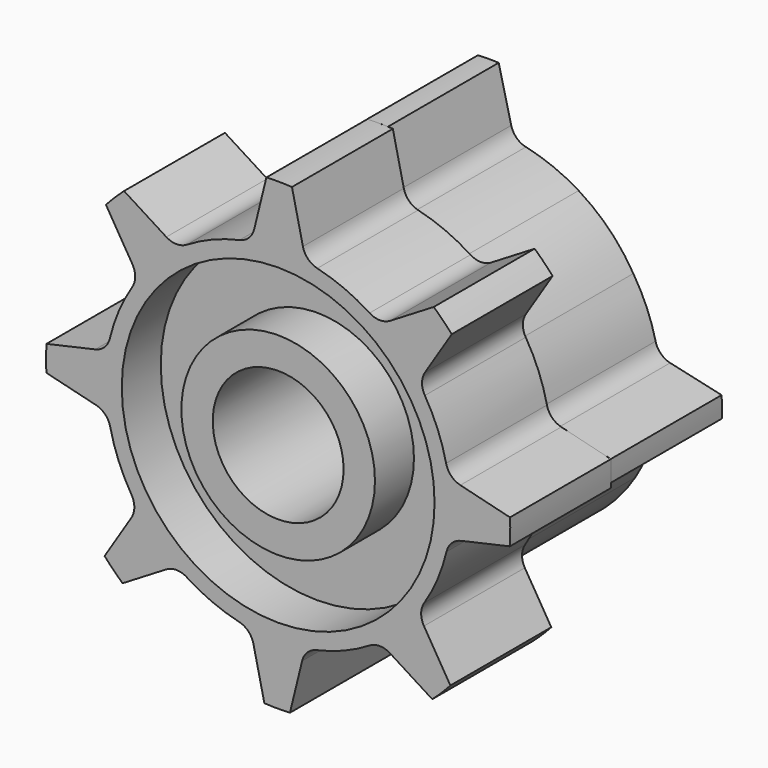
from build123d import *

# Parameters (mm, degrees)
F0_R     = 76.2109388573
F0_R_2   = 51.3540335205
F1_DEPTH = 41.402
F0_R_3   = 31.7840451581
F0_R_4   = 21.4823406774
F2_DEPTH = 25.4
F4_DEPTH = 71.882
F5_DEPTH = 45.466
F6_DEPTH = 31.496
F8_DEPTH = 51.054


with BuildPart() as f1:
    # F0 (on Front) → F1 (new body)
    with BuildSketch(Plane.XZ):
        Circle(F0_R)
        Circle(F0_R_2, mode=Mode.SUBTRACT)
    extrude(amount=F1_DEPTH)

    # F3 (on face) → F4 (cut)
    with BuildSketch(Plane.XZ.offset(41.402)):
        with BuildLine():
            Line((-47.8672647572, 36.7388077798), (-56.5527223926, 51.0871489857))
            ThreePointArc((-56.5527223926, 51.0871489857), (-70.2816834344, 29.4718878788), (-76.0762226062, 4.529410059))
            Line((-76.0762226062, 4.529410059), (-60.0498225812, 8.1337879145))
            ThreePointArc((-60.0498225812, 8.1337879145), (-56.9862917555, 9.8058862302), (-55.2691454533, 12.8443961405))
            ThreePointArc((-55.2691454533, 12.8443961405), (-52.3275453278, 21.741673907), (-47.9509285541, 30.0277941433))
            ThreePointArc((-47.9509285541, 30.0277941433), (-46.9500267793, 33.3713445818), (-47.8672647572, 36.7388077798))
        make_face()
        with BuildLine():
            Line((-7.8690073929, 59.8255276205), (-3.8647440191, 76.1128829777))
            ThreePointArc((-3.8647440191, 76.1128829777), (-28.8568831762, 70.5364267231), (-50.5912363244, 56.9967894593))
            Line((-50.5912363244, 56.9967894593), (-36.7101801652, 48.2130933472))
            ThreePointArc((-36.7101801652, 48.2130933472), (-33.361584686, 47.2292019839), (-29.9988279292, 48.1635471516))
            ThreePointArc((-29.9988279292, 48.1635471516), (-21.6274770901, 52.3748471981), (-12.673569882, 55.1392836076))
            ThreePointArc((-12.673569882, 55.1392836076), (-9.6015782614, 56.7957863637), (-7.8690073929, 59.8255276205))
        make_face()
        with BuildLine():
            ThreePointArc((51.0871489857, 56.5527223926), (29.4718878788, 70.2816834344), (4.529410059, 76.0762226062))
            Line((4.529410059, 76.0762226062), (8.1337879145, 60.0498225812))
            ThreePointArc((8.1337879145, 60.0498225812), (9.8058862302, 56.9862917555), (12.8443961405, 55.2691454533))
            ThreePointArc((12.8443961405, 55.2691454533), (21.741673907, 52.3275453278), (30.0277941433, 47.9509285541))
            ThreePointArc((30.0277941433, 47.9509285541), (33.3713445818, 46.9500267793), (36.7388077798, 47.8672647572))
            Line((36.7388077798, 47.8672647572), (51.0871489857, 56.5527223926))
        make_face()
        with BuildLine():
            ThreePointArc((76.1128829777, 3.8647440191), (70.5364267231, 28.8568831762), (56.9967894593, 50.5912363244))
            Line((56.9967894593, 50.5912363244), (48.2130933472, 36.7101801652))
            ThreePointArc((48.2130933472, 36.7101801652), (47.2292019839, 33.361584686), (48.1635471516, 29.9988279292))
            ThreePointArc((48.1635471516, 29.9988279292), (52.3748471981, 21.6274770901), (55.1392836076, 12.673569882))
            ThreePointArc((55.1392836076, 12.673569882), (56.7957863637, 9.6015782614), (59.8255276205, 7.8690073929))
            Line((59.8255276205, 7.8690073929), (76.1128829777, 3.8647440191))
        make_face()
        with BuildLine():
            ThreePointArc((56.5527223926, -51.0871489857), (70.2816834344, -29.4718878788), (76.0762226062, -4.529410059))
            Line((76.0762226062, -4.529410059), (60.0498225812, -8.1337879145))
            ThreePointArc((60.0498225812, -8.1337879145), (56.9862917555, -9.8058862302), (55.2691454533, -12.8443961405))
            ThreePointArc((55.2691454533, -12.8443961405), (52.3275453278, -21.741673907), (47.9509285541, -30.0277941433))
            ThreePointArc((47.9509285541, -30.0277941433), (46.9500267793, -33.3713445818), (47.8672647572, -36.7388077798))
            Line((47.8672647572, -36.7388077798), (56.5527223926, -51.0871489857))
        make_face()
        with BuildLine():
            ThreePointArc((3.8647440191, -76.1128829777), (28.8568831762, -70.5364267231), (50.5912363244, -56.9967894593))
            Line((50.5912363244, -56.9967894593), (36.7101801652, -48.2130933472))
            ThreePointArc((36.7101801652, -48.2130933472), (33.361584686, -47.2292019839), (29.9988279292, -48.1635471516))
            ThreePointArc((29.9988279292, -48.1635471516), (21.6274770901, -52.3748471981), (12.673569882, -55.1392836076))
            ThreePointArc((12.673569882, -55.1392836076), (9.6015782614, -56.7957863637), (7.8690073929, -59.8255276205))
            Line((7.8690073929, -59.8255276205), (3.8647440191, -76.1128829777))
        make_face()
        with BuildLine():
            Line((-36.7388077798, -47.8672647572), (-51.0871489857, -56.5527223926))
            ThreePointArc((-51.0871489857, -56.5527223926), (-29.4718878788, -70.2816834344), (-4.529410059, -76.0762226062))
            Line((-4.529410059, -76.0762226062), (-8.1337879145, -60.0498225812))
            ThreePointArc((-8.1337879145, -60.0498225812), (-9.8058862302, -56.9862917555), (-12.8443961405, -55.2691454533))
            ThreePointArc((-12.8443961405, -55.2691454533), (-21.741673907, -52.3275453278), (-30.0277941433, -47.9509285541))
            ThreePointArc((-30.0277941433, -47.9509285541), (-33.3713445818, -46.9500267793), (-36.7388077798, -47.8672647572))
        make_face()
        with BuildLine():
            Line((-59.8255276205, -7.8690073929), (-76.1128829777, -3.8647440191))
            ThreePointArc((-76.1128829777, -3.8647440191), (-70.5364267231, -28.8568831762), (-56.9967894593, -50.5912363244))
            Line((-56.9967894593, -50.5912363244), (-48.2130933472, -36.7101801652))
            ThreePointArc((-48.2130933472, -36.7101801652), (-47.2292019839, -33.361584686), (-48.1635471516, -29.9988279292))
            ThreePointArc((-48.1635471516, -29.9988279292), (-52.3748471981, -21.6274770901), (-55.1392836076, -12.673569882))
            ThreePointArc((-55.1392836076, -12.673569882), (-56.7957863637, -9.6015782614), (-59.8255276205, -7.8690073929))
        make_face()
    extrude(amount=-F4_DEPTH, mode=Mode.SUBTRACT)


with BuildPart() as f1b:
    # F0 (on Front) → F1, piece 2 (new body)
    with BuildSketch(Plane.XZ):
        Circle(F0_R_3)
        Circle(F0_R_4, mode=Mode.SUBTRACT)
    extrude(amount=F1_DEPTH)


with BuildPart() as f2:
    # F0 (on Front) → F2 (new body)
    with BuildSketch(Plane.XZ):
        Circle(F0_R_2)
        Circle(F0_R_3, mode=Mode.SUBTRACT)
    extrude(amount=F2_DEPTH)


with BuildPart() as f5:
    # F0 (on Front) → F5 (new body)
    with BuildSketch(Plane.XZ):
        Circle(F0_R_3)
        Circle(F0_R_4, mode=Mode.SUBTRACT)
    extrude(amount=-F5_DEPTH)


with BuildPart() as f5b:
    # F0 (on Front) → F5, piece 2 (new body)
    with BuildSketch(Plane.XZ):
        Circle(F0_R)
        Circle(F0_R_2, mode=Mode.SUBTRACT)
    extrude(amount=-F5_DEPTH)

    # F7 (on face) → F8 (cut)
    with BuildSketch(Plane(origin=(0, 45.466, 0), x_dir=(-1, 0, 0), z_dir=(0, 1, 0))):
        with BuildLine():
            ThreePointArc((-47.1182366423, 29.5992543095), (-39.2509800473, 39.7646962899), (-29.1661360175, 47.7350073178))
            ThreePointArc((-29.1661360175, 47.7350073178), (-20.7947851783, 51.9463073643), (-11.8408779702, 54.7107437738))
            ThreePointArc((-11.8408779702, 54.7107437738), (-8.7688863497, 56.3672465299), (-7.0363154811, 59.3969877867))
            Line((-7.0363154811, 59.3969877867), (-2.9163110774, 76.1551201903))
            ThreePointArc((-2.9163110774, 76.1551201903), (-53.5379377777, 54.2383298048), (-76.1107860532, 3.9058223039))
            Line((-76.1107860532, 3.9058223039), (-59.2171306694, 7.7052480807))
            ThreePointArc((-59.2171306694, 7.7052480807), (-56.1535998437, 9.3773463964), (-54.4364535416, 12.4158563067))
            ThreePointArc((-54.4364535416, 12.4158563067), (-51.494853416, 21.3131340732), (-47.1182366423, 29.5992543095))
        make_face()
        with BuildLine():
            ThreePointArc((76.1551201903, 2.9163110774), (54.2383298048, 53.5379377777), (3.9058223039, 76.1107860532))
            Line((3.9058223039, 76.1107860532), (7.7052480807, 59.2171306694))
            ThreePointArc((7.7052480807, 59.2171306694), (9.3773463964, 56.1535998437), (12.4158563067, 54.4364535416))
            ThreePointArc((12.4158563067, 54.4364535416), (21.3131340732, 51.494853416), (29.5992543095, 47.1182366423))
            ThreePointArc((29.5992543095, 47.1182366423), (39.7646962899, 39.2509800473), (47.7350073178, 29.1661360175))
            ThreePointArc((47.7350073178, 29.1661360175), (51.9463073643, 20.7947851783), (54.7107437738, 11.8408779702))
            ThreePointArc((54.7107437738, 11.8408779702), (56.3672465299, 8.7688863497), (59.3969877867, 7.0363154811))
            Line((59.3969877867, 7.0363154811), (76.1551201903, 2.9163110774))
        make_face()
        with BuildLine():
            ThreePointArc((2.9163110774, -76.1551201903), (53.5379377777, -54.2383298048), (76.1107860532, -3.9058223039))
            Line((76.1107860532, -3.9058223039), (59.2171306694, -7.7052480807))
            ThreePointArc((59.2171306694, -7.7052480807), (56.1535998437, -9.3773463964), (54.4364535416, -12.4158563067))
            ThreePointArc((54.4364535416, -12.4158563067), (51.494853416, -21.3131340732), (47.1182366423, -29.5992543095))
            ThreePointArc((47.1182366423, -29.5992543095), (39.2509800473, -39.7646962899), (29.1661360175, -47.7350073178))
            ThreePointArc((29.1661360175, -47.7350073178), (20.7947851783, -51.9463073643), (11.8408779702, -54.7107437738))
            ThreePointArc((11.8408779702, -54.7107437738), (8.7688863497, -56.3672465299), (7.0363154811, -59.3969877867))
            Line((7.0363154811, -59.3969877867), (2.9163110774, -76.1551201903))
        make_face()
        with BuildLine():
            Line((-59.3969877867, -7.0363154811), (-76.1551201903, -2.9163110774))
            ThreePointArc((-76.1551201903, -2.9163110774), (-54.2383298048, -53.5379377777), (-3.9058223039, -76.1107860532))
            Line((-3.9058223039, -76.1107860532), (-7.7052480807, -59.2171306694))
            ThreePointArc((-7.7052480807, -59.2171306694), (-9.3773463964, -56.1535998437), (-12.4158563067, -54.4364535416))
            ThreePointArc((-12.4158563067, -54.4364535416), (-21.3131340732, -51.494853416), (-29.5992543095, -47.1182366423))
            ThreePointArc((-29.5992543095, -47.1182366423), (-39.7646962899, -39.2509800473), (-47.7350073178, -29.1661360175))
            ThreePointArc((-47.7350073178, -29.1661360175), (-51.9463073643, -20.7947851783), (-54.7107437738, -11.8408779702))
            ThreePointArc((-54.7107437738, -11.8408779702), (-56.3672465299, -8.7688863497), (-59.3969877867, -7.0363154811))
        make_face()
    extrude(amount=-F8_DEPTH, mode=Mode.SUBTRACT)


with BuildPart() as f6:
    # F0 (on Front) → F6 (new body)
    with BuildSketch(Plane.XZ):
        Circle(F0_R_2)
        Circle(F0_R_3, mode=Mode.SUBTRACT)
    extrude(amount=-F6_DEPTH)


solid = Compound([f1.part, f1b.part, f2.part, f5.part, f5b.part, f6.part])
